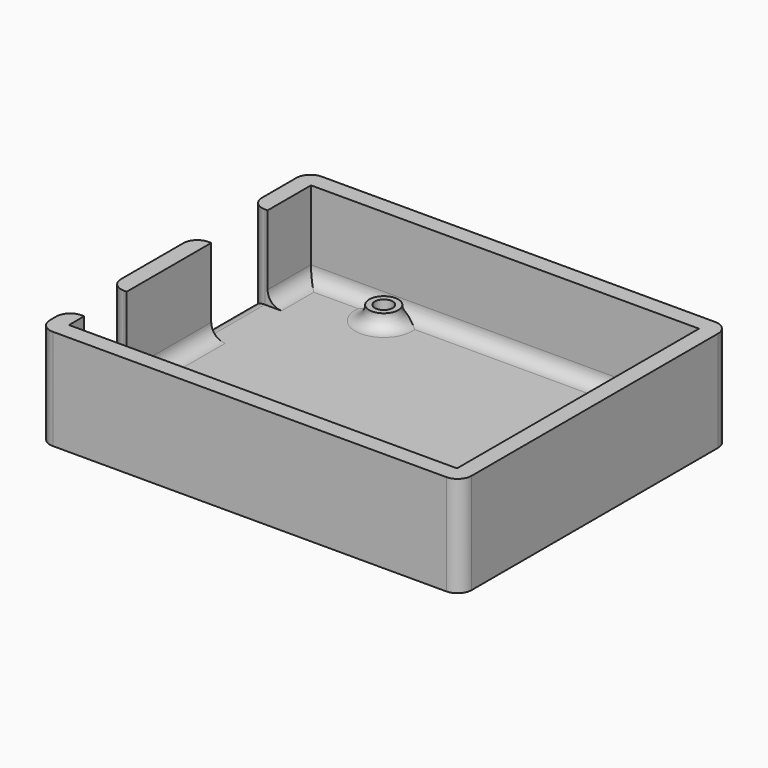
from build123d import *

# Parameters (mm, degrees)
F0_W         = 0.4
F0_H         = 0.3
F0_H_2       = 8.9
F0_W_2       = 9.5
F0_R         = 2.6
F0_W_3       = 10.3
F0_H_3       = 12
F0_W_4       = 3
F0_R_2       = 1.6
F0_H_4       = 18.9
F1_DEPTH     = 3
F2_DEPTH     = 15
F3_DEPTH     = 2.5
F4_T1_DEPTH  = 9.7
F4_T3_DEPTH  = 18.9
F4_T5_DEPTH  = 3.4
F4_T10_DEPTH = 69.4
F4_S11_R     = 2.6
F4_T12_DEPTH = 36
F4_T16_DEPTH = 69.4
F4_S17_R     = 2.6
F4_T18_DEPTH = 36
F4_T22_DEPTH = 54.1
F4_S23_R     = 2.6
F4_T24_DEPTH = 29
F4_S25_R     = 2.6
F4_T26_DEPTH = 29
F4_T35_DEPTH = 30.5
F4_T37_DEPTH = 21.25
F4_T39_DEPTH = 12.6
F4_T41_DEPTH = 9.5
F4_T47_DEPTH = 15.75
F4_T51_DEPTH = 21.25
F4_T59_DEPTH = 18.85
F4_T63_DEPTH = 21.25
F4_T71_DEPTH = 21.25
F4_T76_DEPTH = 18.85
F4_T83_DEPTH = 21.25
F4_T88_DEPTH = 15.75


# Not quite as in the source:
# - a fillet or chamfer that OpenCascade refuses, or shapes differently, is made with other operations: its cross-section is extruded or revolved along the edge and cut away or added


with BuildPart() as f1:
    # F0 (on Top) → F1 (new body)
    with BuildSketch(Plane.XY):
        Polygon((-34.7, -27.05), (-34.7, -23.65), (-37.7, -23.65), (-37.7, -30.05), (37.7, -30.05), (37.7, 30.05), (-37.7, 30.05), (-37.7, 17.35), (-34.7, 17.35), (-34.7, 27.05), (34.7, 27.05), (34.7, -27.05), align=None)
        with Locations((-34.5, -14.3)):
            Rectangle(F0_W, F0_H)
        with Locations((-34.5, -18.9)):
            Rectangle(F0_W, F0_H_2)
        with Locations((-29.55, -18.9)):
            Rectangle(F0_W_2, F0_H_2)
        Polygon((-34.3, -26.65), (34.3, -26.65), (34.3, 26.65), (-34.3, 26.65), (-34.3, 17.35), (-23.7, 17.35), (-23.7, 4.75), (-34.3, 4.75), (-34.3, -14.15), (-24.5, -14.15), (-24.5, -23.65), (-34.3, -23.65), align=None)
        with Locations((-20.3, -23.85)):
            Circle(F0_R, mode=Mode.SUBTRACT)
        with Locations((31.6, -19.15)):
            Circle(F0_R, mode=Mode.SUBTRACT)
        with Locations((-19.2, 23.95)):
            Circle(F0_R, mode=Mode.SUBTRACT)
        with Locations((31.6, 8.75)):
            Circle(F0_R, mode=Mode.SUBTRACT)
        Polygon((34.3, 26.65), (34.3, -26.65), (-34.3, -26.65), (-34.3, -23.65), (-34.7, -23.65), (-34.7, -27.05), (34.7, -27.05), (34.7, 27.05), (-34.7, 27.05), (-34.7, 17.35), (-34.3, 17.35), (-34.3, 26.65), align=None)
        with Locations((-29.15, 11.05)):
            Rectangle(F0_W_3, F0_H_3)
        with Locations((-36.2, 11.05)):
            Rectangle(F0_W_4, F0_H_3)
        with Locations((-34.5, 11.05)):
            Rectangle(F0_W, F0_H_3)
        with Locations((-36.2, -18.9)):
            Rectangle(F0_W_4, F0_H_2)
        with Locations((-36.2, -14.3)):
            Rectangle(F0_W_4, F0_H)
        with Locations((-19.2, 23.95)):
            Circle(F0_R)
        with Locations((-19.2, 23.95)):
            Circle(F0_R_2, mode=Mode.SUBTRACT)
        with Locations((-20.3, -23.85)):
            Circle(F0_R)
        with Locations((-20.3, -23.85)):
            Circle(F0_R_2, mode=Mode.SUBTRACT)
        with Locations((31.6, -19.15)):
            Circle(F0_R)
        with Locations((31.6, -19.15)):
            Circle(F0_R_2, mode=Mode.SUBTRACT)
        with Locations((31.6, 8.75)):
            Circle(F0_R)
        with Locations((31.6, 8.75)):
            Circle(F0_R_2, mode=Mode.SUBTRACT)
        with Locations((-36.2, 4.9)):
            Rectangle(F0_W_4, F0_H)
        with Locations((-34.5, 4.9)):
            Rectangle(F0_W, F0_H)
        Polygon((-23.7, 17.35), (-34.3, 17.35), (-34.3, 17.05), (-24, 17.05), (-24, 5.05), (-34.3, 5.05), (-34.3, 4.75), (-23.7, 4.75), align=None)
        with Locations((-34.5, -4.7)):
            Rectangle(F0_W, F0_H_4)
        with Locations((-36.2, -4.7)):
            Rectangle(F0_W_4, F0_H_4)
        Polygon((-34.3, -23.35), (-34.3, -23.65), (-24.5, -23.65), (-24.5, -14.15), (-34.3, -14.15), (-34.3, -14.45), (-24.8, -14.45), (-24.8, -23.35), align=None)
        with Locations((-36.2, 17.2)):
            Rectangle(F0_W_4, F0_H)
        with Locations((-34.5, 17.2)):
            Rectangle(F0_W, F0_H)
        with Locations((-34.5, -23.5)):
            Rectangle(F0_W, F0_H)
        with Locations((-36.2, -23.5)):
            Rectangle(F0_W_4, F0_H)
    extrude(amount=-F1_DEPTH)

    # F0 (on Top) → F2 (join)
    with BuildSketch(Plane.XY):
        Polygon((-34.7, -27.05), (-34.7, -23.65), (-37.7, -23.65), (-37.7, -30.05), (37.7, -30.05), (37.7, 30.05), (-37.7, 30.05), (-37.7, 17.35), (-34.7, 17.35), (-34.7, 27.05), (34.7, 27.05), (34.7, -27.05), align=None)
        with Locations((-36.2, -4.7)):
            Rectangle(F0_W_4, F0_H_4)
    extrude(amount=F2_DEPTH)

    # F0 (on Top) → F3 (join)
    with BuildSketch(Plane.XY):
        with Locations((-20.3, -23.85)):
            Circle(F0_R)
        with Locations((-20.3, -23.85)):
            Circle(F0_R_2, mode=Mode.SUBTRACT)
        with Locations((-19.2, 23.95)):
            Circle(F0_R)
        with Locations((-19.2, 23.95)):
            Circle(F0_R_2, mode=Mode.SUBTRACT)
        with Locations((31.6, 8.75)):
            Circle(F0_R)
        with Locations((31.6, 8.75)):
            Circle(F0_R_2, mode=Mode.SUBTRACT)
        with Locations((31.6, -19.15)):
            Circle(F0_R)
        with Locations((31.6, -19.15)):
            Circle(F0_R_2, mode=Mode.SUBTRACT)
    extrude(amount=F3_DEPTH)

    # F4: fillet of radius 2.5 on 20 edges, made by hand

    # F4_s2 → F4_t1 (join)
    with BuildSketch(Plane.XZ.offset(-27.05)):
        with BuildLine():
            ThreePointArc((-34.7, 2.5), (-33.967766953, 0.732233047), (-32.2, 0))
            Line((-32.2, 0), (-34.7, 0))
            Line((-34.7, 0), (-34.7, 2.5))
        make_face()
    extrude(amount=F4_T1_DEPTH)

    # F4_s4 → F4_t3 (join)
    with BuildSketch(Plane.XZ.offset(-4.75)):
        with BuildLine():
            ThreePointArc((-32.2, 0), (-33.967766953, 0.732233047), (-34.7, 2.5))
            Line((-34.7, 2.5), (-34.7, 0))
            Line((-34.7, 0), (-32.2, 0))
        make_face()
    extrude(amount=F4_T3_DEPTH)

    # F4_s6 → F4_t5 (join)
    with BuildSketch(Plane.XZ.offset(23.65)):
        with BuildLine():
            ThreePointArc((-34.7, 2.5), (-33.967766953, 0.732233047), (-32.2, 0))
            Line((-32.2, 0), (-34.7, 0))
            Line((-34.7, 0), (-34.7, 2.5))
        make_face()
    extrude(amount=F4_T5_DEPTH)


with BuildPart() as f4_tool8:
    # F4_s9 → F4_t10 (new body)
    with BuildSketch(Plane.YZ.offset(-34.7)):
        with BuildLine():
            ThreePointArc((27.05, 2.5), (26.317766953, 0.732233047), (24.55, 0))
            Line((24.55, 0), (27.05, 0))
            Line((27.05, 0), (27.05, 2.5))
        make_face()
    extrude(amount=F4_T10_DEPTH)

    # F4_s11 → F4_t12 (cut, symmetric)
    with BuildSketch(Plane.XY.offset(1.2)):
        with Locations((-19.2, 23.95)):
            Circle(F4_S11_R)
    extrude(amount=F4_T12_DEPTH, both=True, mode=Mode.SUBTRACT)


with BuildPart() as f1_1:
    add(f1.part)

    # F4_t7: union F4_tool8
    add(f4_tool8.part)


with BuildPart() as f4_tool14:
    # F4_s15 → F4_t16 (new body)
    with BuildSketch(Plane.YZ.offset(34.7)):
        with BuildLine():
            ThreePointArc((-27.05, 2.5), (-26.317766953, 0.732233047), (-24.55, 0))
            Line((-24.55, 0), (-27.05, 0))
            Line((-27.05, 0), (-27.05, 2.5))
        make_face()
    extrude(amount=-F4_T16_DEPTH)

    # F4_s17 → F4_t18 (cut, symmetric)
    with BuildSketch(Plane.XY.offset(1.2)):
        with Locations((-20.3, -23.85)):
            Circle(F4_S17_R)
    extrude(amount=F4_T18_DEPTH, both=True, mode=Mode.SUBTRACT)


with BuildPart() as f1_2:
    add(f1_1.part)

    # F4_t13: union F4_tool14
    add(f4_tool14.part)


with BuildPart() as f4_tool20:
    # F4_s21 → F4_t22 (new body)
    with BuildSketch(Plane.XZ.offset(-27.05)):
        with BuildLine():
            ThreePointArc((34.7, 2.5), (33.967766953, 0.732233047), (32.2, 0))
            Line((32.2, 0), (34.7, 0))
            Line((34.7, 0), (34.7, 2.5))
        make_face()
    extrude(amount=F4_T22_DEPTH)

    # F4_s23 → F4_t24 (cut, symmetric)
    with BuildSketch(Plane.XY.offset(1.2)):
        with Locations((31.6, -19.15)):
            Circle(F4_S23_R)
    extrude(amount=F4_T24_DEPTH, both=True, mode=Mode.SUBTRACT)

    # F4_s25 → F4_t26 (cut, symmetric)
    with BuildSketch(Plane.XY.offset(1.2)):
        with Locations((31.6, 8.75)):
            Circle(F4_S25_R)
    extrude(amount=F4_T26_DEPTH, both=True, mode=Mode.SUBTRACT)


with BuildPart() as f1_3:
    add(f1_2.part)

    # F4_t19: union F4_tool20
    add(f4_tool20.part)

    # F4_s27 → F4_t28 (revolve)
    with BuildSketch(Plane.XZ.offset(-8.75)):
        with BuildLine():
            ThreePointArc((36.7, 0), (34.932233047, 0.732233047), (34.2, 2.5))
            Line((34.2, 2.5), (34.2, 0))
            Line((34.2, 0), (36.7, 0))
        make_face()
    revolve(axis=Axis((31.6, 8.75, 0), (0, 0, 1)))

    # F4_s29 → F4_t30 (revolve)
    with BuildSketch(Plane.XZ.offset(19.15)):
        with BuildLine():
            ThreePointArc((36.7, 0), (34.932233047, 0.732233047), (34.2, 2.5))
            Line((34.2, 2.5), (34.2, 0))
            Line((34.2, 0), (36.7, 0))
        make_face()
    revolve(axis=Axis((31.6, -19.15, 0), (0, 0, 1)))

    # F4_s31 → F4_t32 (revolve)
    with BuildSketch(Plane.XZ.offset(23.85)):
        with BuildLine():
            ThreePointArc((-15.2, 0), (-16.967766953, 0.732233047), (-17.7, 2.5))
            Line((-17.7, 2.5), (-17.7, 0))
            Line((-17.7, 0), (-15.2, 0))
        make_face()
    revolve(axis=Axis((-20.3, -23.85, 0), (0, 0, 1)))

    # F4_s33 → F4_t34 (revolve)
    with BuildSketch(Plane.XZ.offset(-23.95)):
        with BuildLine():
            ThreePointArc((-14.1, 0), (-15.867766953, 0.732233047), (-16.6, 2.5))
            Line((-16.6, 2.5), (-16.6, 0))
            Line((-16.6, 0), (-14.1, 0))
        make_face()
    revolve(axis=Axis((-19.2, 23.95, 0), (0, 0, 1)))

    # F4_s36 → F4_t35 (cut)
    with BuildSketch(Plane.XY.offset(-9.25)):
        with BuildLine():
            ThreePointArc((35.2, -30.05), (36.967766953, -29.317766953), (37.7, -27.55))
            Line((37.7, -27.55), (37.7, -30.05))
            Line((37.7, -30.05), (35.2, -30.05))
        make_face()
        with BuildLine():
            ThreePointArc((37.7, 27.55), (36.967766953, 29.317766953), (35.2, 30.05))
            Line((35.2, 30.05), (37.7, 30.05))
            Line((37.7, 30.05), (37.7, 27.55))
        make_face()
        with BuildLine():
            ThreePointArc((-37.7, 27.55), (-36.967766953, 29.317766953), (-35.2, 30.05))
            Line((-35.2, 30.05), (-37.7, 30.05))
            Line((-37.7, 30.05), (-37.7, 27.55))
        make_face()
        with BuildLine():
            ThreePointArc((-35.2, -30.05), (-36.967766953, -29.317766953), (-37.7, -27.55))
            Line((-37.7, -27.55), (-37.7, -30.05))
            Line((-37.7, -30.05), (-35.2, -30.05))
        make_face()
    extrude(amount=F4_T35_DEPTH, mode=Mode.SUBTRACT)

    # F4_s38 → F4_t37 (cut)
    with BuildSketch(Plane.XY):
        with BuildLine():
            ThreePointArc((-37.7, -11.65), (-36.967766953, -13.417766953), (-35.2, -14.15))
            Line((-35.2, -14.15), (-37.7, -14.15))
            Line((-37.7, -14.15), (-37.7, -11.65))
        make_face()
        with BuildLine():
            ThreePointArc((-37.7, 19.85), (-36.967766953, 18.082233047), (-35.2, 17.35))
            Line((-35.2, 17.35), (-37.7, 17.35))
            Line((-37.7, 17.35), (-37.7, 19.85))
        make_face()
        with BuildLine():
            ThreePointArc((-37.7, 2.25), (-36.967766953, 4.017766953), (-35.2, 4.75))
            Line((-35.2, 4.75), (-37.7, 4.75))
            Line((-37.7, 4.75), (-37.7, 2.25))
        make_face()
        with BuildLine():
            ThreePointArc((-37.7, -26.15), (-36.967766953, -24.382233047), (-35.2, -23.65))
            Line((-35.2, -23.65), (-37.7, -23.65))
            Line((-37.7, -23.65), (-37.7, -26.15))
        make_face()
    extrude(amount=F4_T37_DEPTH, mode=Mode.SUBTRACT)

    # F4_s40 → F4_t39 (cut)
    with BuildSketch(Plane.XZ.offset(-17.35)):
        with BuildLine():
            ThreePointArc((-37.7, -2.5), (-36.967766953, -0.732233047), (-35.2, 0))
            Line((-35.2, 0), (-37.7, 0))
            Line((-37.7, 0), (-37.7, -2.5))
        make_face()
    extrude(amount=F4_T39_DEPTH, mode=Mode.SUBTRACT)

    # F4_s42 → F4_t41 (cut)
    with BuildSketch(Plane.XZ.offset(14.15)):
        with BuildLine():
            ThreePointArc((-37.7, -2.5), (-36.967766953, -0.732233047), (-35.2, 0))
            Line((-35.2, 0), (-37.7, 0))
            Line((-37.7, 0), (-37.7, -2.5))
        make_face()
    extrude(amount=F4_T41_DEPTH, mode=Mode.SUBTRACT)


with BuildPart() as f4_tool45:
    # F4_s46 → F4_t47 (new body)
    with BuildSketch(Plane.XZ.offset(7.9)):
        with BuildLine():
            ThreePointArc((-37.7, -2.5), (-36.967766953, -0.732233047), (-35.2, 0))
            Line((-35.2, 0), (-37.7, 0))
            Line((-37.7, 0), (-37.7, -2.5))
        make_face()
    extrude(amount=F4_T47_DEPTH)

    split(bisect_by=Plane.XZ.offset(14.15), keep=Keep.BOTTOM)


with BuildPart() as f4_tool49:
    # F4_s50 → F4_t51 (new body)
    with BuildSketch(Plane.XY.offset(-6.25)):
        with BuildLine():
            ThreePointArc((-37.7, -11.65), (-36.967766953, -13.417766953), (-35.2, -14.15))
            Line((-35.2, -14.15), (-37.7, -14.15))
            Line((-37.7, -14.15), (-37.7, -11.65))
        make_face()
    extrude(amount=F4_T51_DEPTH)

    split(bisect_by=Plane.XY.offset(-3), keep=Keep.TOP)

    split(bisect_by=Plane.XY, keep=Keep.BOTTOM)


with BuildPart() as f4_tool45_1:
    add(f4_tool45.part)

    # F4_t54: intersect F4_tool49
    add(f4_tool49.part, mode=Mode.INTERSECT)


with BuildPart() as f1_4:
    add(f1_3.part)

    # F4_t43: cut F4_tool45
    add(f4_tool45_1.part, mode=Mode.SUBTRACT)


with BuildPart() as f4_tool57:
    # F4_s58 → F4_t59 (new body)
    with BuildSketch(Plane.XZ.offset(-23.6)):
        with BuildLine():
            ThreePointArc((-37.7, -2.5), (-36.967766953, -0.732233047), (-35.2, 0))
            Line((-35.2, 0), (-37.7, 0))
            Line((-37.7, 0), (-37.7, -2.5))
        make_face()
    extrude(amount=F4_T59_DEPTH)

    split(bisect_by=Plane.XZ.offset(-17.35), keep=Keep.BOTTOM)


with BuildPart() as f4_tool61:
    # F4_s62 → F4_t63 (new body)
    with BuildSketch(Plane.XY.offset(-6.25)):
        with BuildLine():
            ThreePointArc((-37.7, 19.85), (-36.967766953, 18.082233047), (-35.2, 17.35))
            Line((-35.2, 17.35), (-37.7, 17.35))
            Line((-37.7, 17.35), (-37.7, 19.85))
        make_face()
    extrude(amount=F4_T63_DEPTH)

    split(bisect_by=Plane.XY.offset(-3), keep=Keep.TOP)

    split(bisect_by=Plane.XY, keep=Keep.BOTTOM)


with BuildPart() as f4_tool57_1:
    add(f4_tool57.part)

    # F4_t66: intersect F4_tool61
    add(f4_tool61.part, mode=Mode.INTERSECT)


with BuildPart() as f1_5:
    add(f1_4.part)

    # F4_t55: cut F4_tool57
    add(f4_tool57_1.part, mode=Mode.SUBTRACT)


with BuildPart() as f4_tool69:
    # F4_s70 → F4_t71 (new body)
    with BuildSketch(Plane.XY.offset(-6.25)):
        with BuildLine():
            ThreePointArc((-37.7, 2.25), (-36.967766953, 4.017766953), (-35.2, 4.75))
            Line((-35.2, 4.75), (-37.7, 4.75))
            Line((-37.7, 4.75), (-37.7, 2.25))
        make_face()
    extrude(amount=F4_T71_DEPTH)

    split(bisect_by=Plane.XY.offset(-3), keep=Keep.TOP)

    split(bisect_by=Plane.XY, keep=Keep.BOTTOM)


with BuildPart() as f4_tool74:
    # F4_s75 → F4_t76 (new body)
    with BuildSketch(Plane.XZ.offset(-17.35)):
        with BuildLine():
            ThreePointArc((-37.7, -2.5), (-36.967766953, -0.732233047), (-35.2, 0))
            Line((-35.2, 0), (-37.7, 0))
            Line((-37.7, 0), (-37.7, -2.5))
        make_face()
    extrude(amount=F4_T76_DEPTH)

    split(bisect_by=Plane.XZ.offset(-4.75), keep=Keep.TOP)


with BuildPart() as f4_tool69_1:
    add(f4_tool69.part)

    # F4_t78: intersect F4_tool74
    add(f4_tool74.part, mode=Mode.INTERSECT)


with BuildPart() as f1_6:
    add(f1_5.part)

    # F4_t67: cut F4_tool69
    add(f4_tool69_1.part, mode=Mode.SUBTRACT)


with BuildPart() as f4_tool81:
    # F4_s82 → F4_t83 (new body)
    with BuildSketch(Plane.XY.offset(-6.25)):
        with BuildLine():
            ThreePointArc((-37.7, -26.15), (-36.967766953, -24.382233047), (-35.2, -23.65))
            Line((-35.2, -23.65), (-37.7, -23.65))
            Line((-37.7, -23.65), (-37.7, -26.15))
        make_face()
    extrude(amount=F4_T83_DEPTH)

    split(bisect_by=Plane.XY.offset(-3), keep=Keep.TOP)

    split(bisect_by=Plane.XY, keep=Keep.BOTTOM)


with BuildPart() as f4_tool86:
    # F4_s87 → F4_t88 (new body)
    with BuildSketch(Plane.XZ.offset(14.15)):
        with BuildLine():
            ThreePointArc((-37.7, -2.5), (-36.967766953, -0.732233047), (-35.2, 0))
            Line((-35.2, 0), (-37.7, 0))
            Line((-37.7, 0), (-37.7, -2.5))
        make_face()
    extrude(amount=F4_T88_DEPTH)

    split(bisect_by=Plane.XZ.offset(23.65), keep=Keep.TOP)


with BuildPart() as f4_tool81_1:
    add(f4_tool81.part)

    # F4_t90: intersect F4_tool86
    add(f4_tool86.part, mode=Mode.INTERSECT)


with BuildPart() as f1_7:
    add(f1_6.part)

    # F4_t79: cut F4_tool81
    add(f4_tool81_1.part, mode=Mode.SUBTRACT)


solid = f1_7.part
